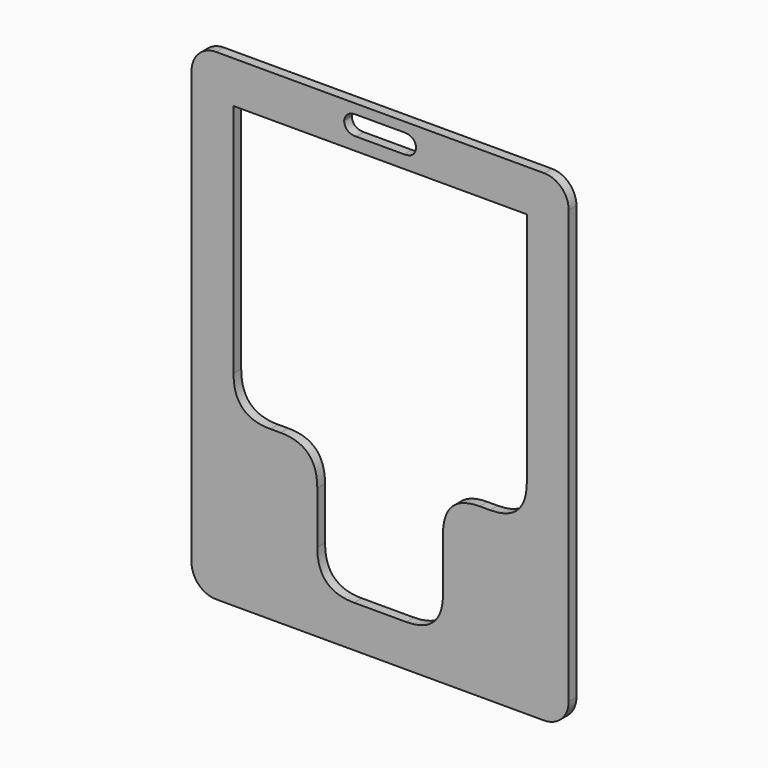
from build123d import *

# Parameters (mm, degrees)
F0_W         = 781.2
F0_H         = 998.2
F1_DEPTH     = 20
F2_R         = 50.8
F4_DEPTH     = 25.4
F5_T1_DEPTH  = 20
F5_T3_DEPTH  = 401
F6_W         = 260.4
F6_H         = 46.8
F7_DEPTH     = 25.4
F8_W         = 150
F8_H         = 40
F9_DEPTH     = 20.0010001
F10_T1_DEPTH = 20


# Not quite as in the source:
# - a fillet or chamfer that OpenCascade refuses, or shapes differently, is made with other operations: its cross-section is extruded or revolved along the edge and cut away or added


with BuildPart() as f1:
    # F0 (on Front) → F1 (new body)
    with BuildSketch(Plane.XZ):
        Rectangle(F0_W, F0_H)
    extrude(amount=F1_DEPTH)

    # F2
    f2_edges = [f1.edges().sort_by_distance(p)[0] for p in [
        (-390.6, -10, 499.1),
        (390.6, -10, 499.1),
        (390.6, -10, -499.1),
        (-390.6, -10, -499.1),
    ]]
    fillet(f2_edges, radius=F2_R)

    # F3 (on Front) → F4 (cut)
    with BuildSketch(Plane.XZ):
        Polygon((303.8, 412.3), (-303.8, 412.3), (-303.8, -151.9), (-130.2, -151.9), (-130.2, -412.3), (130.2, -412.3), (130.2, -151.9), (303.8, -151.9), align=None)
    extrude(amount=F4_DEPTH, mode=Mode.SUBTRACT)

    # F5: fillet of radius 76.2 on 6 edges, made by hand

    # F5_s2 → F5_t1 (join)
    with BuildSketch(Plane.XZ):
        with BuildLine():
            add(Edge.make_bspline(
                [(-303.8, -75.7), (-303.8, -151.9), (-227.6, -151.9)],
                knots=[0, 0, 0, 1, 1, 1], degree=2, weights=[1, 1, 1]))
            Line((-227.6, -151.9), (-303.8, -151.9))
            Line((-303.8, -151.9), (-303.8, -75.7))
        make_face()
        with BuildLine():
            add(Edge.make_bspline(
                [(-130.2, -336.1), (-130.2, -412.3), (-54, -412.3)],
                knots=[0, 0, 0, 1, 1, 1], degree=2, weights=[1, 1, 1]))
            Line((-54, -412.3), (-130.2, -412.3))
            Line((-130.2, -412.3), (-130.2, -336.1))
        make_face()
        with BuildLine():
            add(Edge.make_bspline(
                [(227.6, -151.9), (303.8, -151.9), (303.8, -75.7)],
                knots=[0, 0, 0, 1, 1, 1], degree=2, weights=[1, 1, 1]))
            Line((303.8, -75.7), (303.8, -151.9))
            Line((303.8, -151.9), (227.6, -151.9))
        make_face()
        with BuildLine():
            add(Edge.make_bspline(
                [(54, -412.3), (130.2, -412.3), (130.2, -336.1)],
                knots=[0, 0, 0, 1, 1, 1], degree=2, weights=[1, 1, 1]))
            Line((130.2, -336.1), (130.2, -412.3))
            Line((130.2, -412.3), (54, -412.3))
        make_face()
    extrude(amount=F5_T1_DEPTH)

    # F5_s4 → F5_t3 (cut)
    with BuildSketch(Plane.XZ.offset(-190.5)):
        with BuildLine():
            add(Edge.make_bspline(
                [(-206.4, -151.9), (-130.2, -151.9), (-130.2, -228.1)],
                knots=[0, 0, 0, 1, 1, 1], degree=2, weights=[1, 1, 1]))
            Line((-130.2, -228.1), (-130.2, -151.9))
            Line((-130.2, -151.9), (-206.4, -151.9))
        make_face()
        with BuildLine():
            add(Edge.make_bspline(
                [(130.2, -228.1), (130.2, -151.9), (206.4, -151.9)],
                knots=[0, 0, 0, 1, 1, 1], degree=2, weights=[1, 1, 1]))
            Line((206.4, -151.9), (130.2, -151.9))
            Line((130.2, -151.9), (130.2, -228.1))
        make_face()
    extrude(amount=F5_T3_DEPTH, mode=Mode.SUBTRACT)

    # F6 (on Front) → F7 (cut)
    with BuildSketch(Plane.XZ):
        with Locations((0, 455.7)):
            Rectangle(F6_W, F6_H)
    extrude(amount=-F7_DEPTH, mode=Mode.SUBTRACT)

    # F8 (on face) → F9 (cut, through all)
    with BuildSketch(Plane.XZ.offset(20)):
        with Locations((0, 459.1)):
            Rectangle(F8_W, F8_H)
    extrude(amount=-F9_DEPTH, mode=Mode.SUBTRACT)

    # F10: fillet of radius 25.4 on 4 edges, made by hand

    # F10_s2 → F10_t1 (join)
    with BuildSketch(Plane.XZ):
        with BuildLine():
            add(Edge.make_bspline(
                [(-49.6, 479.1), (-75, 479.1), (-75, 453.7)],
                knots=[0, 0, 0, 1, 1, 1], degree=2, weights=[1, 1, 1]))
            Line((-75, 453.7), (-75, 479.1))
            Line((-75, 479.1), (-49.6, 479.1))
        make_face()
        with BuildLine():
            add(Edge.make_bspline(
                [(-75, 464.5), (-75, 439.1), (-49.6, 439.1)],
                knots=[0, 0, 0, 1, 1, 1], degree=2, weights=[1, 1, 1]))
            Line((-49.6, 439.1), (-75, 439.1))
            Line((-75, 439.1), (-75, 464.5))
        make_face()
        with BuildLine():
            add(Edge.make_bspline(
                [(49.6, 479.1), (75, 479.1), (75, 453.7)],
                knots=[0, 0, 0, 1, 1, 1], degree=2, weights=[1, 1, 1]))
            Line((75, 453.7), (75, 479.1))
            Line((75, 479.1), (49.6, 479.1))
        make_face()
        with BuildLine():
            add(Edge.make_bspline(
                [(49.6, 439.1), (75, 439.1), (75, 464.5)],
                knots=[0, 0, 0, 1, 1, 1], degree=2, weights=[1, 1, 1]))
            Line((75, 464.5), (75, 439.1))
            Line((75, 439.1), (49.6, 439.1))
        make_face()
    extrude(amount=F10_T1_DEPTH)


solid = f1.part
